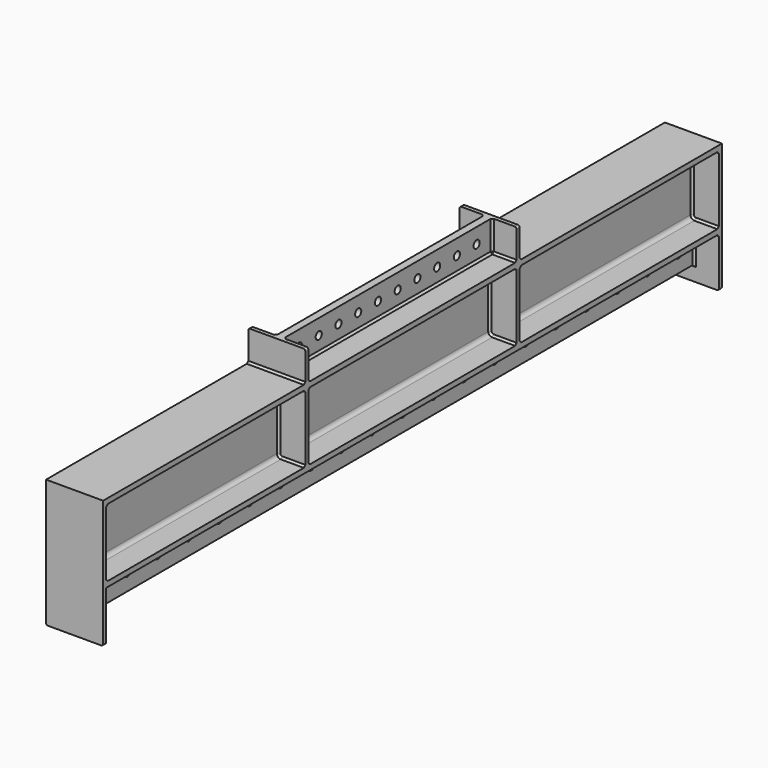
from build123d import *

# Parameters (mm, degrees)
F1_DEPTH      = 2540
F2_W          = 863.6
F2_H          = 101.6
F2_R          = 12.7
F3_DEPTH      = 12.7
F3_DEPTH_BACK = 12.7
F4_W          = 2540
F4_H          = 114.3
F4_R          = 14.2875
F5_DEPTH      = 12.7
F5_DEPTH_BACK = 12.7
F6_W          = 81.915
F6_H          = 114.3
F7_DEPTH      = 12.7
F8_W          = 189.23
F8_H          = 373.888
F9_DEPTH      = 12.7
F10_W         = 189.23
F10_H         = 101.6
F10_W_2       = 81.915
F11_DEPTH     = 12.7
F13_DEPTH     = 12.7
F14_W         = 189.23
F14_H         = 12.7
F15_DEPTH     = 50.8
F16_W         = 12.7
F16_H         = 225.044
F17_DEPTH     = 189.23
F18_R         = 6.35
F19_R         = 6.35
F20_SIZE      = 6.35


with BuildPart() as f1:
    # F0 (on Front) → F1 (new body)
    with BuildSketch(Plane.XZ):
        with BuildLine():
            Line((94.615, 259.588), (-94.615, 259.588))
            Line((-94.615, 259.588), (-94.615, 242.316))
            Line((-94.615, 242.316), (-18.2245, 242.316))
            ThreePointArc((-18.2245, 242.316), (-9.1095400371, 238.5404599629), (-5.334, 229.4255))
            Line((-5.334, 229.4255), (-5.334, 30.1625))
            ThreePointArc((-5.334, 30.1625), (-9.1095400371, 21.0475400371), (-18.2245, 17.272))
            Line((-18.2245, 17.272), (-94.615, 17.272))
            Line((-94.615, 17.272), (-94.615, 0))
            Line((-94.615, 0), (94.615, 0))
            Line((94.615, 0), (94.615, 17.272))
            Line((94.615, 17.272), (18.2245, 17.272))
            ThreePointArc((18.2245, 17.272), (9.1095400371, 21.0475400371), (5.334, 30.1625))
            Line((5.334, 30.1625), (5.334, 229.4255))
            ThreePointArc((5.334, 229.4255), (9.1095400371, 238.5404599629), (18.2245, 242.316))
            Line((18.2245, 242.316), (94.615, 242.316))
            Line((94.615, 242.316), (94.615, 259.588))
        make_face()
    extrude(amount=F1_DEPTH)

    # F2 (on Right) → F3 (join, two sides)
    with BuildSketch(Plane.YZ) as f3_sk:
        with Locations((-1270, 310.388)):
            Rectangle(F2_W, F2_H)
        with Locations((-1638.29999492, 310.388)):
            Circle(F2_R, mode=Mode.SUBTRACT)
        with Locations((-1556.45555104, 310.388)):
            Circle(F2_R, mode=Mode.SUBTRACT)
        with Locations((-1474.61110716, 310.388)):
            Circle(F2_R, mode=Mode.SUBTRACT)
        with Locations((-1392.76666328, 310.388)):
            Circle(F2_R, mode=Mode.SUBTRACT)
        with Locations((-1310.9222194, 310.388)):
            Circle(F2_R, mode=Mode.SUBTRACT)
        with Locations((-1229.07777552, 310.388)):
            Circle(F2_R, mode=Mode.SUBTRACT)
        with Locations((-1147.23333164, 310.388)):
            Circle(F2_R, mode=Mode.SUBTRACT)
        with Locations((-1065.38888776, 310.388)):
            Circle(F2_R, mode=Mode.SUBTRACT)
        with Locations((-983.54444388, 310.388)):
            Circle(F2_R, mode=Mode.SUBTRACT)
        with Locations((-901.7, 310.388)):
            Circle(F2_R, mode=Mode.SUBTRACT)
    extrude(amount=F3_DEPTH)
    extrude(f3_sk.sketch, amount=-F3_DEPTH_BACK)

    # F4 (on Right) → F5 (join, two sides)
    with BuildSketch(Plane.YZ) as f5_sk:
        with Locations((-1270, -57.15)):
            Rectangle(F4_W, F4_H)
        with Locations((-2476.5, -57.15)):
            Circle(F4_R, mode=Mode.SUBTRACT)
        with Locations((-2349.5, -57.15)):
            Circle(F4_R, mode=Mode.SUBTRACT)
        with Locations((-2222.5, -57.15)):
            Circle(F4_R, mode=Mode.SUBTRACT)
        with Locations((-2095.5, -57.15)):
            Circle(F4_R, mode=Mode.SUBTRACT)
        with Locations((-1968.5, -57.15)):
            Circle(F4_R, mode=Mode.SUBTRACT)
        with Locations((-1841.5, -57.15)):
            Circle(F4_R, mode=Mode.SUBTRACT)
        with Locations((-1714.5, -57.15)):
            Circle(F4_R, mode=Mode.SUBTRACT)
        with Locations((-1587.5, -57.15)):
            Circle(F4_R, mode=Mode.SUBTRACT)
        with Locations((-1460.5, -57.15)):
            Circle(F4_R, mode=Mode.SUBTRACT)
        with Locations((-1333.5, -57.15)):
            Circle(F4_R, mode=Mode.SUBTRACT)
        with Locations((-1206.5, -57.15)):
            Circle(F4_R, mode=Mode.SUBTRACT)
        with Locations((-1079.5, -57.15)):
            Circle(F4_R, mode=Mode.SUBTRACT)
        with Locations((-952.5, -57.15)):
            Circle(F4_R, mode=Mode.SUBTRACT)
        with Locations((-825.5, -57.15)):
            Circle(F4_R, mode=Mode.SUBTRACT)
        with Locations((-698.5, -57.15)):
            Circle(F4_R, mode=Mode.SUBTRACT)
        with Locations((-571.5, -57.15)):
            Circle(F4_R, mode=Mode.SUBTRACT)
        with Locations((-444.5, -57.15)):
            Circle(F4_R, mode=Mode.SUBTRACT)
        with Locations((-317.5, -57.15)):
            Circle(F4_R, mode=Mode.SUBTRACT)
        with Locations((-190.5, -57.15)):
            Circle(F4_R, mode=Mode.SUBTRACT)
        with Locations((-63.5, -57.15)):
            Circle(F4_R, mode=Mode.SUBTRACT)
    extrude(amount=F5_DEPTH)
    extrude(f5_sk.sketch, amount=-F5_DEPTH_BACK)

    # F6 (on face) → F7 (join)
    with BuildSketch(Plane(origin=(0, 0, 0), x_dir=(-1, 0, 0), z_dir=(0, 1, 0))):
        with Locations((53.6575, -57.15)):
            Rectangle(F6_W, F6_H)
        with BuildLine():
            Line((-18.2245, 242.316), (-94.615, 242.316))
            Line((-94.615, 242.316), (-94.615, 17.272))
            Line((-94.615, 17.272), (-18.2245, 17.272))
            ThreePointArc((-18.2245, 17.272), (-9.1095400371, 21.0475400371), (-5.334, 30.1625))
            Line((-5.334, 30.1625), (-5.334, 229.4255))
            ThreePointArc((-5.334, 229.4255), (-9.1095400371, 238.5404599629), (-18.2245, 242.316))
        make_face()
        with BuildLine():
            Line((94.615, 17.272), (94.615, 242.316))
            Line((94.615, 242.316), (18.2245, 242.316))
            ThreePointArc((18.2245, 242.316), (9.1095400371, 238.5404599629), (5.334, 229.4255))
            Line((5.334, 229.4255), (5.334, 30.1625))
            ThreePointArc((5.334, 30.1625), (9.1095400371, 21.0475400371), (18.2245, 17.272))
            Line((18.2245, 17.272), (94.615, 17.272))
        make_face()
        with BuildLine():
            Line((94.615, 259.588), (-94.615, 259.588))
            Line((-94.615, 259.588), (-94.615, 242.316))
            Line((-94.615, 242.316), (-18.2245, 242.316))
            ThreePointArc((-18.2245, 242.316), (-9.1095400371, 238.5404599629), (-5.334, 229.4255))
            Line((-5.334, 229.4255), (-5.334, 30.1625))
            ThreePointArc((-5.334, 30.1625), (-9.1095400371, 21.0475400371), (-18.2245, 17.272))
            Line((-18.2245, 17.272), (-94.615, 17.272))
            Line((-94.615, 17.272), (-94.615, 0))
            Line((-94.615, 0), (-12.7, 0))
            Line((-12.7, 0), (-12.7, -114.3))
            Line((-12.7, -114.3), (12.7, -114.3))
            Line((12.7, -114.3), (12.7, 0))
            Line((12.7, 0), (94.615, 0))
            Line((94.615, 0), (94.615, 17.272))
            Line((94.615, 17.272), (18.2245, 17.272))
            ThreePointArc((18.2245, 17.272), (9.1095400371, 21.0475400371), (5.334, 30.1625))
            Line((5.334, 30.1625), (5.334, 229.4255))
            ThreePointArc((5.334, 229.4255), (9.1095400371, 238.5404599629), (18.2245, 242.316))
            Line((18.2245, 242.316), (94.615, 242.316))
            Line((94.615, 242.316), (94.615, 259.588))
        make_face()
        with Locations((-53.6575, -57.15)):
            Rectangle(F6_W, F6_H)
    extrude(amount=F7_DEPTH)

    # F8 (on face) → F9 (join)
    with BuildSketch(Plane.XZ.offset(2540)):
        with Locations((0, 72.644)):
            Rectangle(F8_W, F8_H)
    extrude(amount=F9_DEPTH)

    # F10 (on face) → F11 (join)
    with BuildSketch(Plane.XZ.offset(1701.8)):
        with Locations((0, 310.388)):
            Rectangle(F10_W, F10_H)
        with Locations((53.6575, 310.388)):
            Rectangle(F10_W_2, F10_H)
    extrude(amount=F11_DEPTH)

    # F12 (on face) → F13 (join)
    with BuildSketch(Plane(origin=(0, -838.2, 0), x_dir=(-1, 0, 0), z_dir=(0, 1, 0))):
        Polygon((-12.7, 259.588), (12.7, 259.588), (94.615, 259.588), (94.615, 361.188), (12.7, 361.188), (-12.7, 361.188), (-94.615, 361.188), (-94.615, 259.588), align=None)
    extrude(amount=F13_DEPTH)

    # F14 (on face) → F15 (join)
    with BuildSketch(Plane(origin=(0, 0, -114.3), x_dir=(1, 0, 0), z_dir=(0, 0, -1))):
        with Locations((0, -6.35)):
            Rectangle(F14_W, F14_H)
        with Locations((0, 2546.35)):
            Rectangle(F14_W, F14_H)
    extrude(amount=F15_DEPTH)

    # F16 (on face) → F17 (join)
    with BuildSketch(Plane.YZ.offset(94.615)):
        with Locations((-1708.15, 129.794)):
            Rectangle(F16_W, F16_H)
        with Locations((-831.85, 129.794)):
            Rectangle(F16_W, F16_H)
    extrude(amount=-F17_DEPTH)

    # F18
    f18_edges = [f1.edges().sort_by_distance(p)[0] for p in [
        (-94.615, -831.85, 361.188),
        (94.615, -831.85, 361.188),
        (94.615, -1708.15, 361.188),
        (-94.615, -1708.15, 361.188),
    ]]
    fillet(f18_edges, radius=F18_R)

    # F19
    f19_edges = [f1.edges().sort_by_distance(p)[0] for p in [
        (94.615, -2546.35, -165.1),
        (-94.615, -2546.35, -165.1),
        (-94.615, 6.35, -165.1),
        (94.615, 6.35, -165.1),
    ]]
    fillet(f19_edges, radius=F19_R)

    # F20
    f20_edges = [f1.edges().sort_by_distance(p)[0] for p in [
        (-12.7, -1270, 0),
        (12.7, -1270, 0),
        (12.7, 0, -57.15),
        (12.7, -2540, -57.15),
        (0, -2540, -114.3),
        (-12.7, -2540, -57.15),
        (0, 0, -114.3),
        (-12.7, 0, -57.15),
        (5.334, 0, 129.794),
        (-53.6575, 0, 0),
        (53.6575, 0, 0),
        (-5.334, 0, 129.794),
        (5.334, -2540, 129.794),
        (-5.334, -2540, 129.794),
        (-56.41975, -1714.5, 17.272),
        (-5.334, -1701.8, 129.794),
        (-5.334, -825.5, 129.794),
        (-5.334, -838.2, 129.794),
        (5.334, -825.5, 129.794),
        (5.334, -838.2, 129.794),
        (5.334, -1714.5, 129.794),
        (5.334, -1701.8, 129.794),
        (53.6575, -1701.8, 259.588),
        (12.7, -1270, 259.588),
        (53.6575, -838.2, 259.588),
        (0, -825.5, 259.588),
        (0, -1714.5, 259.588),
        (12.7, -1701.8, 310.388),
        (12.7, -838.2, 310.388),
        (-12.7, -1270, 259.588),
        (-53.6575, -1701.8, 259.588),
        (-12.7, -1701.8, 310.388),
        (-53.6575, -838.2, 259.588),
        (-12.7, -838.2, 310.388),
    ]]
    chamfer(f20_edges, length=F20_SIZE)


solid = f1.part
